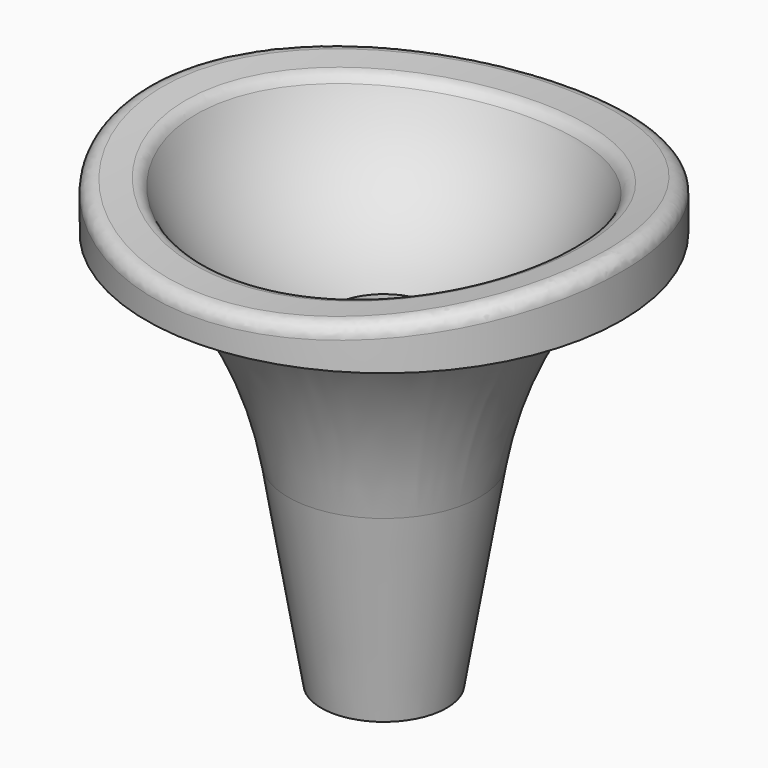
from build123d import *

# Parameters (mm, degrees)
F3_DEPTH      = 34.9237274141
F3_DEPTH_BACK = 34.9237274141
F4_R          = 2


with BuildPart() as f1:
    # F0 (on Front) → F1 (revolve)
    with BuildSketch(Plane.XZ):
        with BuildLine():
            Line((7.7161088216, 46.5042699361), (7.2837931816, 0))
            Line((7.2837931816, 0), (9.2186463284, 0))
            Line((9.2186463284, 0), (14.0412328462, 28.8096964042))
            ThreePointArc((14.0412328462, 28.8096964042), (19.0762362079, 44.660996201), (28.3428626439, 58.4720279725))
            Line((28.3428626439, 58.4720279725), (34.9227274141, 58.4720279725))
            Line((34.9227274141, 58.4720279725), (34.9227274141, 67.2027245164))
            Line((34.9227274141, 67.2027245164), (28.275898718, 67.2027245164))
            ThreePointArc((28.275898718, 67.2027245164), (20.7596401025, 54.1083752592), (7.7161088216, 46.5042699361))
        make_face()
    revolve(axis=Axis((0, 0, 29.2033459991), (0, 0, 1)))

    # F2 (on Front) → F3 (cut, two sides)
    with BuildSketch(Plane.XZ) as f3_sk:
        with BuildLine():
            Line((34.9227274141, 67.2027245164), (-34.9227274141, 67.2027245164))
            ThreePointArc((-34.9227274141, 67.2027245164), (0, 63.7732244017), (34.9227274141, 67.2027245164))
        make_face()
    extrude(amount=-F3_DEPTH, mode=Mode.SUBTRACT)
    extrude(f3_sk.sketch, amount=F3_DEPTH_BACK, mode=Mode.SUBTRACT)

    # F4
    f4_edges = [f1.edges().sort_by_distance(p)[0] for p in [
        (-27.91449, 0, 65.956733),
        (1e-06, 34.922727, 63.773224),
        (1e-06, -34.922727, 63.773224),
    ]]
    fillet(f4_edges, radius=F4_R)


solid = f1.part
